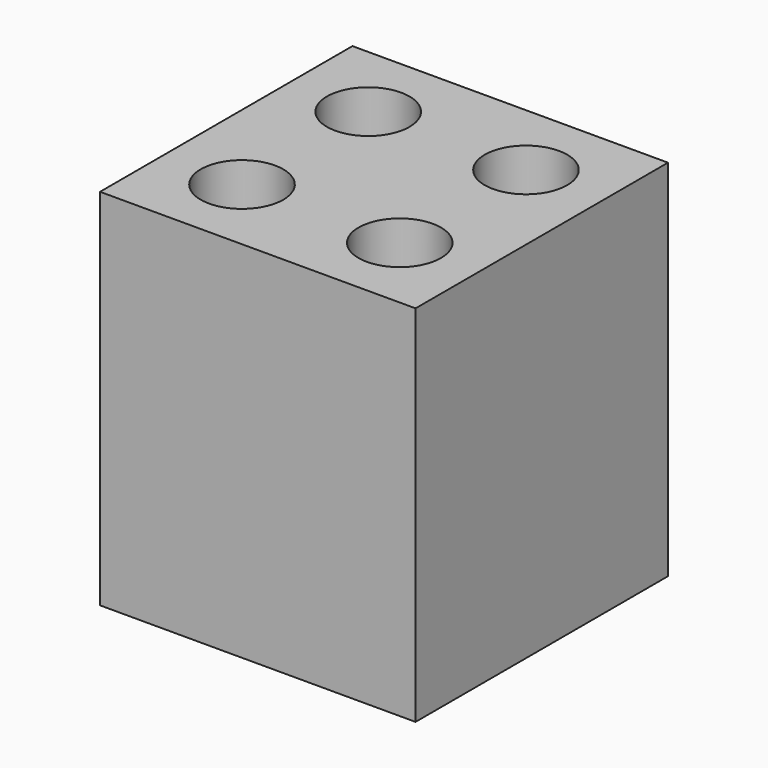
from build123d import *

# Parameters (mm, degrees)
F0_W        = 65
F0_H        = 65
F0_R        = 8.5
F1_DEPTH    = 75
F2_T        = -1.778
F3_T1_DEPTH = 61.444
F3_T3_DEPTH = 61.444


# Not quite as in the source:
# - a fillet or chamfer that OpenCascade refuses, or shapes differently, is made with other operations: its cross-section is extruded or revolved along the edge and cut away or added


with BuildPart() as f1:
    # F0 (on Top) → F1 (new body)
    with BuildSketch(Plane.XY):
        Rectangle(F0_W, F0_H)
        with Locations((-16.25, -16.25)):
            Circle(F0_R, mode=Mode.SUBTRACT)
        with Locations((16.25, -16.25)):
            Circle(F0_R, mode=Mode.SUBTRACT)
        with Locations((-16.25, 16.25)):
            Circle(F0_R, mode=Mode.SUBTRACT)
        with Locations((16.25, 16.25)):
            Circle(F0_R, mode=Mode.SUBTRACT)
    extrude(amount=F1_DEPTH)

    # F2
    f2_openings = [f1.faces().sort_by_distance(p)[0] for p in [
        (0, 0, 0),
    ]]
    offset(amount=F2_T, openings=f2_openings)

    # F3: fillet of radius 5.08 on 8 edges, made by hand

    # F3_s2 → F3_t1 (join)
    with BuildSketch(Plane.YZ.offset(-30.722)):
        with BuildLine():
            ThreePointArc((30.722, 68.142), (29.2341024484, 71.7341024484), (25.642, 73.222))
            Line((25.642, 73.222), (30.722, 73.222))
            Line((30.722, 73.222), (30.722, 68.142))
        make_face()
        with BuildLine():
            ThreePointArc((-30.722, 68.142), (-29.2341024484, 71.7341024484), (-25.642, 73.222))
            Line((-25.642, 73.222), (-30.722, 73.222))
            Line((-30.722, 73.222), (-30.722, 68.142))
        make_face()
    extrude(amount=F3_T1_DEPTH)

    # F3_s4 → F3_t3 (join)
    with BuildSketch(Plane.XZ.offset(-30.722)):
        with BuildLine():
            ThreePointArc((-30.722, 68.142), (-29.2341024484, 71.7341024484), (-25.642, 73.222))
            Line((-25.642, 73.222), (-30.722, 73.222))
            Line((-30.722, 73.222), (-30.722, 68.142))
        make_face()
        with BuildLine():
            ThreePointArc((30.722, 68.142), (29.2341024484, 71.7341024484), (25.642, 73.222))
            Line((25.642, 73.222), (30.722, 73.222))
            Line((30.722, 73.222), (30.722, 68.142))
        make_face()
    extrude(amount=F3_T3_DEPTH)

    # F3_s5 → F3_t6 (revolve)
    with BuildSketch(Plane.XZ.offset(16.25)):
        with BuildLine():
            ThreePointArc((-0.892, 73.222), (-4.4841024484, 71.7341024484), (-5.972, 68.142))
            Line((-5.972, 68.142), (-5.972, 73.222))
            Line((-5.972, 73.222), (-0.892, 73.222))
        make_face()
    revolve(axis=Axis((-16.25, -16.25, 73.222), (0, 0, -1)))

    # F3_s7 → F3_t8 (revolve)
    with BuildSketch(Plane.XZ.offset(16.25)):
        with BuildLine():
            ThreePointArc((31.608, 73.222), (28.0158975516, 71.7341024484), (26.528, 68.142))
            Line((26.528, 68.142), (26.528, 73.222))
            Line((26.528, 73.222), (31.608, 73.222))
        make_face()
    revolve(axis=Axis((16.25, -16.25, 73.222), (0, 0, -1)))

    # F3_s9 → F3_t10 (revolve)
    with BuildSketch(Plane.XZ.offset(-16.25)):
        with BuildLine():
            ThreePointArc((-0.892, 73.222), (-4.4841024484, 71.7341024484), (-5.972, 68.142))
            Line((-5.972, 68.142), (-5.972, 73.222))
            Line((-5.972, 73.222), (-0.892, 73.222))
        make_face()
    revolve(axis=Axis((-16.25, 16.25, 73.222), (0, 0, -1)))

    # F3_s11 → F3_t12 (revolve)
    with BuildSketch(Plane.XZ.offset(-16.25)):
        with BuildLine():
            ThreePointArc((31.608, 73.222), (28.0158975516, 71.7341024484), (26.528, 68.142))
            Line((26.528, 68.142), (26.528, 73.222))
            Line((26.528, 73.222), (31.608, 73.222))
        make_face()
    revolve(axis=Axis((16.25, 16.25, 73.222), (0, 0, -1)))


solid = f1.part
